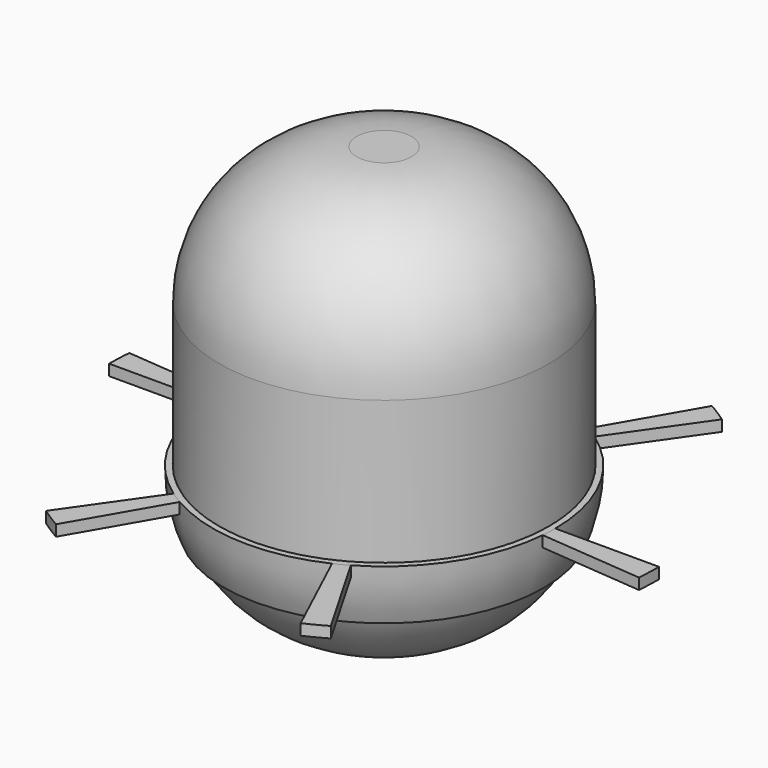
from build123d import *

# Parameters (mm, degrees)
F2_R     = 25
F3_R     = 25
F7_E36_W = 18.8636766477
F7_E36_H = 2
F7_E35_W = 18.8636344634
F7_E35_H = 2
F7_E38_W = 18.863644271
F7_E38_H = 2
F7_E39_W = 18.863644271
F7_E39_H = 2
F7_E40_W = 18.8636344634
F7_E40_H = 2
F7_E37_W = 18.8636766477
F7_E37_H = 2
F8_ANGLE = 5


with BuildPart() as f1:
    # F0 (on Front) → F1 (revolve)
    with BuildSketch(Plane.XZ):
        with BuildLine():
            add(Edge.make_bspline(
                [(0, 45.4371280968), (-3.0004580163, 44.9671513003), (-9.2125643156, 45.4390536746), (-16.5528259828, 38.4439243544), (-21.0979577111, 32.6096007506), (-25.5305000368, 23.423243266), (-27.6968929758, 13.5818536342), (-27.8185750233, 8.5768682772), (-27.6943626983, 5.6445188447), (-27.6821504659, 5.3903233737)],
                knots=[0, 0, 0, 0, 0.0910944553, 0.1843060983, 0.2679290185, 0.3646805118, 0.4608654522, 0.5438819223, 0.5516533593, 0.5516533593, 0.5516533593, 0.5516533593], degree=3))
            Line((0, 45.4371280968), (0, 48.4371280968))
            Line((0, 48.4371280968), (-30, 48.4371280968))
            Line((-30, 48.4371280968), (-30, 48.2053891704))
            Line((-30, 48.2053891704), (-30, 5.3903233737))
            Line((-30, 5.3903233737), (-27.6821504659, 5.3903233737))
        make_face()
        with BuildLine():
            add(Edge.make_bspline(
                [(-27.6821504659, 5.3903233737), (-27.6358761265, 4.42713114), (-27.5669211006, 3.4181859016), (-27.4624139886, 2.390275872)],
                knots=[0.5516533593, 0.5516533593, 0.5516533593, 0.5516533593, 0.5811007281, 0.5811007281, 0.5811007281, 0.5811007281], degree=3))
            Line((-27.6821504659, 5.3903233737), (-30, 5.3903233737))
            Line((-30, 5.3903233737), (-30, 2.390275872))
            Line((-30, 2.390275872), (-27.4624139886, 2.390275872))
        make_face()
        with BuildLine():
            Line((0, -27.5628719032), (0, -24.5628719032))
            add(Edge.make_bspline(
                [(-27.4624139886, 2.390275872), (-27.2510669776, 0.3115110068), (-26.3372358046, -5.212057084), (-22.2963186711, -12.42136403), (-16.3834656207, -18.253014288), (-6.6944776159, -22.7949319845), (-2.1106013755, -24.494400447), (0, -24.5628719032)],
                knots=[0.5811007281, 0.5811007281, 0.5811007281, 0.5811007281, 0.640652784, 0.7336471032, 0.8212898622, 0.9204482508, 1, 1, 1, 1], degree=3))
            Line((-27.4624139886, 2.390275872), (-30, 2.390275872))
            Line((-30, 2.390275872), (-30, -21.7946108296))
            Line((-30, -21.7946108296), (-30, -27.5628719032))
            Line((-30, -27.5628719032), (0, -27.5628719032))
        make_face()
    revolve(axis=Axis((0, 0, 10.4371280968), (0, 0, -1)))

    # F2
    f2_edges = [f1.edges().sort_by_distance(p)[0] for p in [
        (30, 0, 48.437128),
    ]]
    fillet(f2_edges, radius=F2_R)

    # F3
    f3_edges = [f1.edges().sort_by_distance(p)[0] for p in [
        (-30, 0, -2.062872),
        (30, 0, 23.437128),
        (30, 0, -27.562872),
    ]]
    fillet(f3_edges, radius=F3_R)


with BuildPart() as f5:
    # F4 (on Front) → F5 (revolve)
    with BuildSketch(Plane.XZ):
        with BuildLine():
            ThreePointArc((29.0602930781, -12.7435246812), (30.6120609744, -7.7579601565), (31.1363655366, -2.5628719032))
            Line((31.1363655366, -2.5628719032), (30.0182903195, -2.5628719032))
            ThreePointArc((30.0182903195, -2.5628719032), (29.4676776295, -7.7683913527), (27.8402086015, -12.7435246812))
            Line((27.8402086015, -12.7435246812), (29.0602930781, -12.7435246812))
        make_face()
    revolve(axis=Axis((0, 0, 10.4371280968), (0, 0, -1)))

    # F7_E36 (on explicit) + F7_E35 (on explicit) + F7_E38 (on explicit) + F7_E39 (on explicit) + F7_E40 (on explicit) + F7_E37 (on explicit) → F8 (revolve)
    with BuildSketch(Plane(origin=(15.5333254356, -26.9849784091, -2.5628719032), x_dir=(0.5, -0.8660254038, 0), z_dir=(0.8660254038, 0.5, 0))):
        with Locations((9.4318383239, 1)):
            Rectangle(F7_E36_W, F7_E36_H)
    with BuildSketch(Plane(origin=(31.1363655366, 0, -2.5628719032), x_dir=(1, 0, 0), z_dir=(0, 1, 0))):
        with Locations((9.4318172317, 1)):
            Rectangle(F7_E35_W, F7_E35_H)
    with BuildSketch(Plane(origin=(15.5333254356, 26.9849784091, -2.5628719032), x_dir=(0.5, 0.8660254038, 0), z_dir=(-0.8660254038, 0.5, 0))):
        with Locations((9.4318221355, 1)):
            Rectangle(F7_E38_W, F7_E38_H)
    with BuildSketch(Plane(origin=(-15.6030141051, 26.944743637, -2.5628719032), x_dir=(-0.5, 0.8660254038, 0), z_dir=(-0.8660254038, -0.5, 0))):
        with Locations((9.4318221355, 1)):
            Rectangle(F7_E39_W, F7_E39_H)
    with BuildSketch(Plane(origin=(-31.1363655366, 0, -2.5628719032), x_dir=(-1, 0, 0), z_dir=(0, -1, 0))):
        with Locations((9.4318172317, 1)):
            Rectangle(F7_E40_W, F7_E40_H)
    with BuildSketch(Plane(origin=(-15.6030141051, -26.944743637, -2.5628719032), x_dir=(-0.5, -0.8660254038, 0), z_dir=(0.8660254038, -0.5, 0))):
        with Locations((9.4318383239, 1)):
            Rectangle(F7_E37_W, F7_E37_H)
    revolve(axis=Axis((0, 0, 10.4371280968), (0, 0, -1)), revolution_arc=F8_ANGLE)


solid = Compound([f1.part, f5.part])
